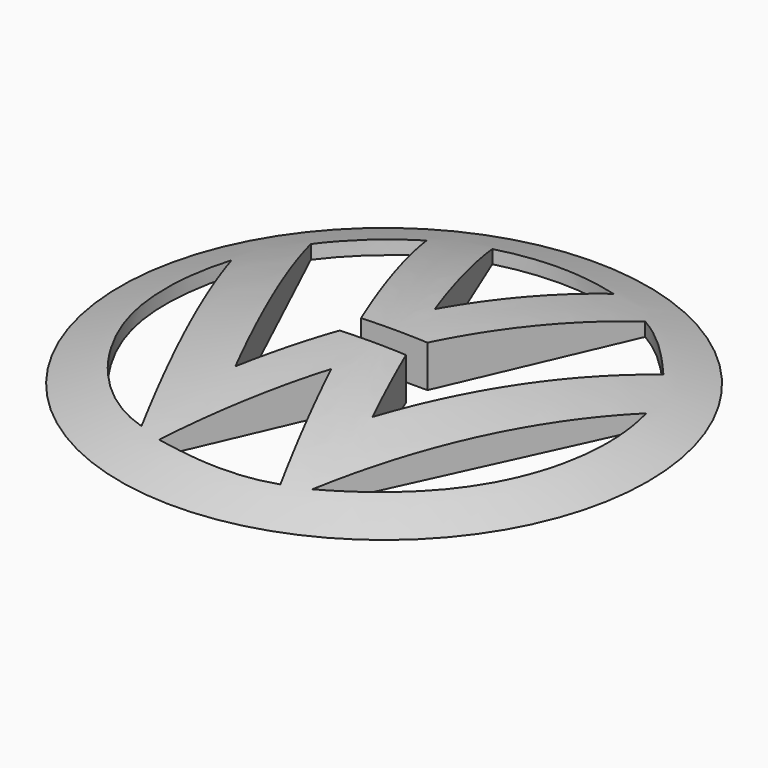
from build123d import *

# Parameters (mm, degrees)
F0_R     = 31
F1_DEPTH = 5


# Not quite as in the source:
# - the dataset's text gives a spline's control points without its knots; the knots are read off the source's solid


with BuildPart() as f1:
    # F0 (on Top) → F1 (new body)
    with BuildSketch(Plane.XY):
        with Locations((0.8609048494, -0.1599287318)):
            Circle(F0_R)
        with BuildLine():
            add(Edge.make_bspline(
                [(-23.488278884, 7.8908103673), (-24.6961455584, 3.6319057668), (-25.3545343956, -3.9042310318), (-20.2970320428, -15.5188133176), (-14.2839209538, -21.5008309202), (-9.1907718286, -23.2125382974)],
                knots=[0, 0, 0, 0, 0.3585793833, 0.5756727949, 1, 1, 1, 1], degree=3))
            Line((-23.488278884, 7.8908103673), (-9.1907718286, -23.2125382974))
        make_face(mode=Mode.SUBTRACT)
        with BuildLine():
            add(Edge.make_bspline(
                [(-6.2488954054, -24.292164956), (-1.5996124574, -25.3234601333), (3.3582465294, -25.8097194051), (7.9831177949, -24.292164956)],
                knots=[0, 0, 0, 0, 1, 1, 1, 1], degree=3))
            Line((-6.2488954054, -24.292164956), (0.8609048494, -7.8974941689))
            Line((0.8609048494, -7.8974941689), (7.9831177949, -24.292164956))
        make_face(mode=Mode.SUBTRACT)
        with BuildLine():
            Line((10.8801437045, -23.2125382974), (25.2066760781, 7.8908103673))
            add(Edge.make_bspline(
                [(25.2066760781, 7.8908103673), (26.5603332217, 3.074549187), (26.5075749111, -4.8659077439), (21.0987271112, -16.2435346498), (15.0674965542, -21.0903552903), (10.8801437045, -23.2125382974)],
                knots=[0, 0, 0, 0, 0.4007768334, 0.6183123162, 1, 1, 1, 1], degree=3))
        make_face(mode=Mode.SUBTRACT)
        with BuildLine():
            Line((-7.2182016156, -11.8989486888), (-19.7968107448, 14.8995758))
            add(Edge.make_bspline(
                [(-19.7968107448, 14.8995758), (-17.6815708766, 17.7818081478), (-14.9583292897, 20.167138439), (-12.0064102931, 22.1588673185)],
                knots=[0, 0, 0, 0, 1, 1, 1, 1], degree=3))
            Line((-12.0064102931, 22.1588673185), (-3.0653384403, 1.3593045285))
            Line((-3.0653384403, 1.3593045285), (4.7351615391, 1.3593045285))
            Line((4.7351615391, 1.3593045285), (13.7230759355, 22.1013271976))
            add(Edge.make_bspline(
                [(13.7230759355, 22.1013271976), (16.8572867392, 20.305723039), (19.2771128834, 17.5803722778), (21.6188905101, 14.8995758)],
                knots=[0, 0, 0, 0, 1, 1, 1, 1], degree=3))
            Line((21.6188905101, 14.8995758), (8.8865023402, -11.8989486888))
            Line((8.8865023402, -11.8989486888), (4.7351615391, -1.7784003418))
            Line((4.7351615391, -1.7784003418), (-3.0653384403, -1.7784003418))
            Line((-3.0653384403, -1.7784003418), (-7.2182016156, -11.8989486888))
        make_face(mode=Mode.SUBTRACT)
        with BuildLine():
            Line((0.8609048494, 7.2844412145), (-6.2488954054, 24.610305664))
            add(Edge.make_bspline(
                [(-6.2488954054, 24.610305664), (-1.608836888, 25.8386968792), (3.3444632423, 25.9224389776), (7.9831177949, 24.610305664)],
                knots=[0, 0, 0, 0, 1, 1, 1, 1], degree=3))
            Line((7.9831177949, 24.610305664), (0.8609048494, 7.2844412145))
        make_face(mode=Mode.SUBTRACT)
    extrude(amount=F1_DEPTH)

    # F4 (on line) → F5 (revolve, cut)
    with BuildSketch(Plane(origin=(0, -0.1599287318, 0), x_dir=(-1, 0, 0), z_dir=(0, 1, 0))):
        with BuildLine():
            ThreePointArc((-31.8609048494, 0), (-16.5612233175, 3.7419745023), (-0.8609048494, 5))
            Line((-0.8609048494, 5), (-0.8609048494, 6.381183397))
            Line((-0.8609048494, 6.381183397), (-31.8609048494, 6.381183397))
            Line((-31.8609048494, 6.381183397), (-31.8609048494, 0))
        make_face()
    revolve(axis=Axis((0.8609048494, -0.1599287318, 5.6905916985), (0, 0, 1)), mode=Mode.SUBTRACT)


solid = f1.part
